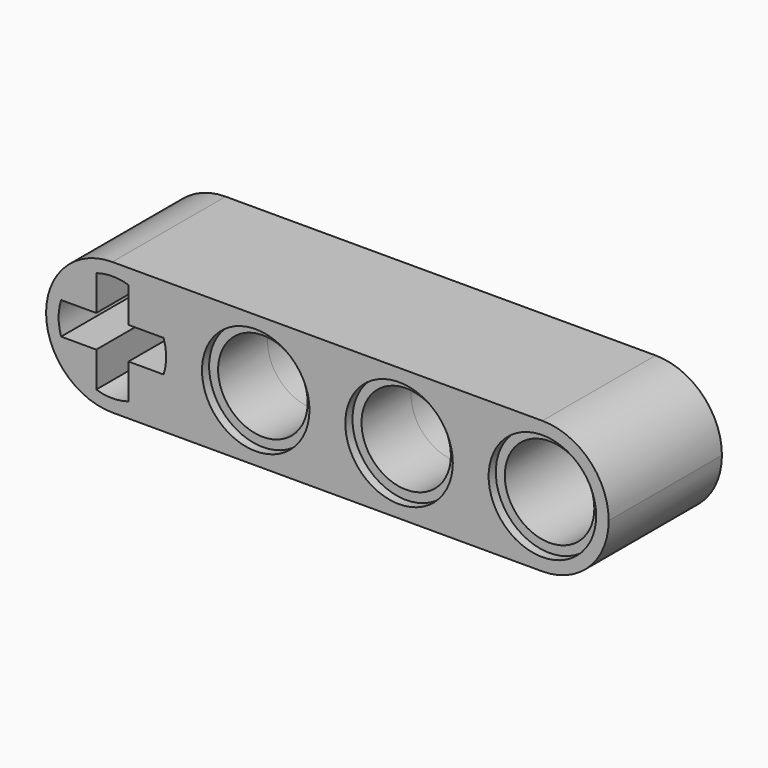
from build123d import *

# Parameters (mm, degrees)
F0_R     = 3
F1_DEPTH = 3.95
F0_R_2   = 2.499
F0_R_3   = 2.495
F2_DEPTH = 3.45
F3_R     = 3.69999


# Not quite as in the source:
# - a fillet or chamfer is up to 0.001 mm smaller than in the source, because OpenCascade refuses the exact size


with BuildPart() as f1:
    # F0 (on Front) → F1 (new body, symmetric)
    with BuildSketch(Plane.XZ):
        Polygon((15.7, -3.7), (15.7, 0), (15.7, 3.7), (-15.7, 3.7), (-15.7, -3.7), align=None)
        with BuildLine():
            ThreePointArc((-12.8998169675, 2.8618751589), (-11.9998409744, 2.9999999958), (-11.0998796299, 2.8617797468))
            Line((-11.0998796299, 2.8617797468), (-11.0998796299, 0.8996879915))
            Line((-11.0998796299, 0.8996879915), (-9.1380842923, 0.8996879915))
            ThreePointArc((-9.1380842923, 0.8996879915), (-9.0000000001, -2.51387e-05), (-9.1380993707, -0.8997359546))
            Line((-9.1380993707, -0.8997359546), (-11.0998796299, -0.8997359546))
            Line((-11.0998796299, -0.8997359546), (-11.0998796299, -2.8617797468))
            ThreePointArc((-11.0998796299, -2.8617797468), (-11.9998409744, -2.9999999958), (-12.8998169675, -2.8618751589))
            Line((-12.8998169675, -2.8618751589), (-12.8998169675, -0.8997359546))
            Line((-12.8998169675, -0.8997359546), (-14.8619006293, -0.8997359546))
            ThreePointArc((-14.8619006293, -0.8997359546), (-14.9999999999, -2.51387e-05), (-14.8619157077, 0.8996879915))
            Line((-14.8619157077, 0.8996879915), (-12.8998169675, 0.8996879915))
            Line((-12.8998169675, 0.8996879915), (-12.8998169675, 2.8618751589))
        make_face(mode=Mode.SUBTRACT)
        with Locations((-4, 0)):
            Circle(F0_R, mode=Mode.SUBTRACT)
        with Locations((4, 0)):
            Circle(F0_R, mode=Mode.SUBTRACT)
        with Locations((12, 0)):
            Circle(F0_R, mode=Mode.SUBTRACT)
    extrude(amount=F1_DEPTH, both=True)

    # F0 (on Front) → F2 (join, symmetric)
    with BuildSketch(Plane.XZ):
        with Locations((-4, 0)):
            Circle(F0_R)
        with Locations((-4, 0)):
            Circle(F0_R_2, mode=Mode.SUBTRACT)
        with Locations((4, 0)):
            Circle(F0_R)
        with Locations((4, 0)):
            Circle(F0_R_3, mode=Mode.SUBTRACT)
        with Locations((12, 0)):
            Circle(F0_R)
        with Locations((12, 0)):
            Circle(F0_R_2, mode=Mode.SUBTRACT)
    extrude(amount=F2_DEPTH, both=True)

    # F3 (radius 3.7 in the source; OpenCascade refuses exactly that, so slightly less here)
    f3_edges = [f1.edges().sort_by_distance(p)[0] for p in [
        (-15.7, 0, 3.7),
        (-15.7, 0, -3.7),
        (15.7, 0, 3.7),
        (15.7, 0, -3.7),
    ]]
    fillet(f3_edges, radius=F3_R)


solid = f1.part
